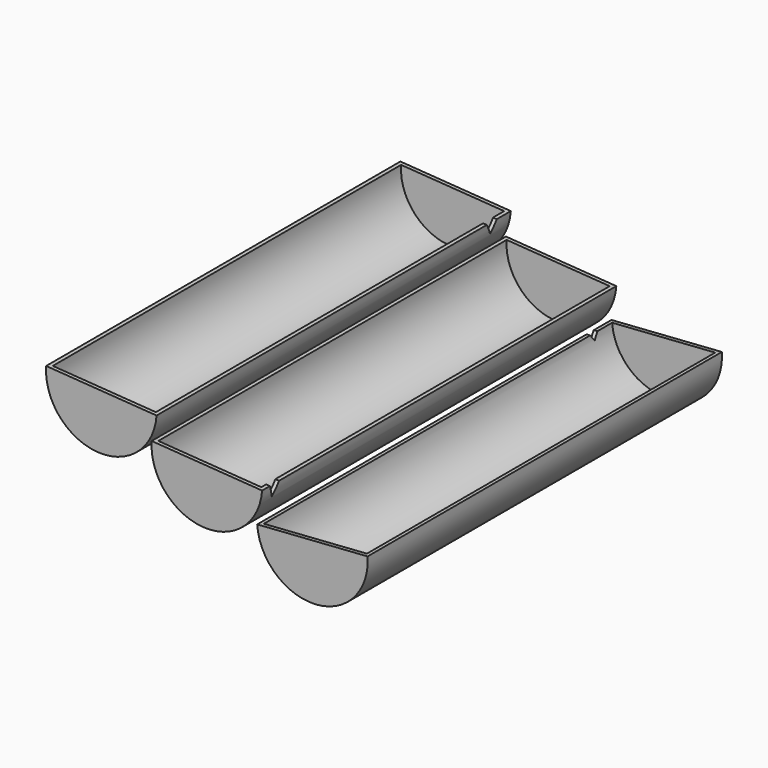
from build123d import *

# Parameters (mm, degrees)
F1_DEPTH  = 600
F3_DEPTH  = 5
F5_DEPTH  = 5
F6_ANGLE  = 4
F10_DEPTH = 178
F13_DEPTH = 121
F16_ANGLE = -8
F17_DEPTH = 105


with BuildPart() as f1:
    # F0 (on Front) → F1 (new body)
    with BuildSketch(Plane.XZ):
        with BuildLine():
            ThreePointArc((-75, 0), (0, -75), (75, 0))
            Line((75, 0), (70, 0))
            ThreePointArc((70, 0), (0, -70), (-70, 0))
            Line((-70, 0), (-75, 0))
        make_face()
    extrude(amount=F1_DEPTH)

    # F2 (on face) → F3 (join)
    with BuildSketch(Plane.XZ.offset(600)):
        with BuildLine():
            Line((70, 0), (-70, 0))
            ThreePointArc((-70, 0), (0, -70), (70, 0))
        make_face()
    extrude(amount=-F3_DEPTH)

    # F4 (on face) → F5 (join)
    with BuildSketch(Plane(origin=(0, 0, 0), x_dir=(-1, 0, 0), z_dir=(0, 1, 0))):
        with BuildLine():
            Line((70, 0), (-70, 0))
            ThreePointArc((-70, 0), (0, -70), (70, 0))
        make_face()
    extrude(amount=-F5_DEPTH)


with BuildPart() as f1_1:
    # F6: moved
    add(f1.part.rotate(Axis((75, -300, 0), (0, 1, 0)), F6_ANGLE))


with BuildPart() as f7_1:
    # F7: copy of F1
    add(f1_1.part.moved(Location((143, 0, -43))))


with BuildPart() as f8_1:
    # F8: copy of F7_1
    add(f7_1.part.moved(Location((143, 0, -53))))


with BuildPart() as f1_2:
    add(f1_1.part)

    # F9 (on Right) → F10 (cut)
    with BuildSketch(Plane.YZ):
        Polygon((-31.8559333682, -15.1517242193), (-18.6419468373, 10.0749731064), (-47.4724583328, 11.8768755347), align=None)
    extrude(amount=F10_DEPTH, mode=Mode.SUBTRACT)


with BuildPart() as f7_1_1:
    add(f7_1.part)

    # F12 (on offset) → F13 (cut)
    with BuildSketch(Plane.YZ.offset(166)):
        Polygon((-569.4248080254, -39.1771495342), (-588.6451601982, -38.5765135288), (-580.193400383, -59.3179017305), align=None)
    extrude(amount=F13_DEPTH, mode=Mode.SUBTRACT)


with BuildPart() as f8_1_1:
    # F16: moved
    add(f8_1.part.rotate(Axis((211.365392461, -300, -85.5365289384), (0, 1, 0)), F16_ANGLE))

    # F15 (on offset) → F17 (cut)
    with BuildSketch(Plane.YZ.offset(316)):
        Polygon((-35.931546241, -93.5071781278), (-15.5054412415, -65.7264964947), (-57.7888276324, -64.9577161884), align=None)
    extrude(amount=-F17_DEPTH, mode=Mode.SUBTRACT)


solid = Compound([f1_2.part, f7_1_1.part, f8_1_1.part])
